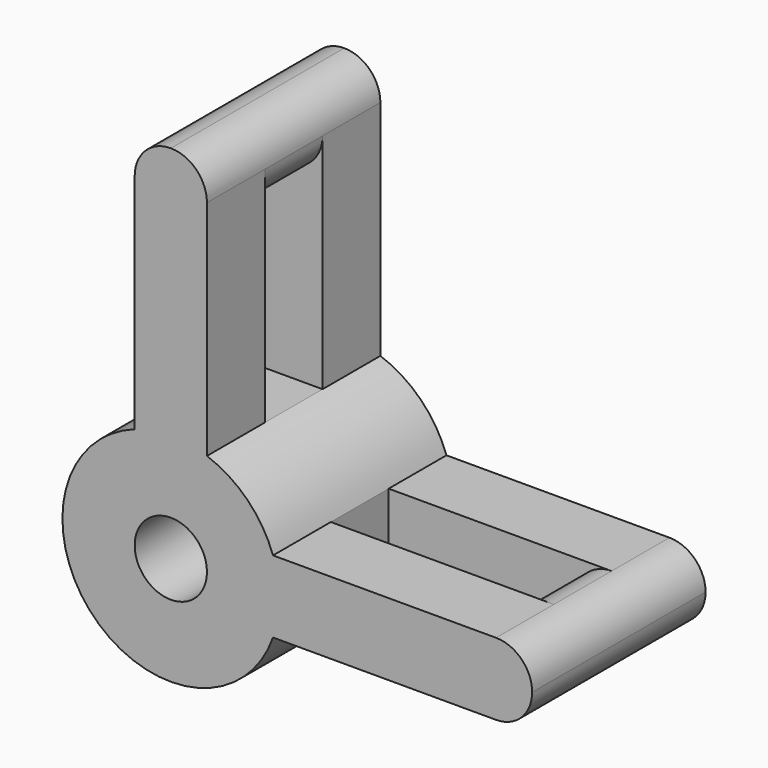
from build123d import *

# Parameters (mm, degrees)
F1_DEPTH = 15
F2_W     = 5
F2_H     = 12.9289321881
F3_DEPTH = 25
F4_W     = 12.9289321881
F4_H     = 5
F5_DEPTH = 25
F6_R     = 2.49999
F7_R     = 2.5
F8_DEPTH = 25


# Not quite as in the source:
# - a fillet or chamfer is up to 0.001 mm smaller than in the source, because OpenCascade refuses the exact size


with BuildPart() as f1:
    # F0 (on Front) → F1 (new body)
    with BuildSketch(Plane.XZ):
        with BuildLine():
            Line((2.5, 25), (-2.5, 25))
            Line((-2.5, 25), (-2.5, 7.0710678119))
            ThreePointArc((-2.5, 7.0710678119), (-5.3033008589, -5.3033008589), (7.0710678119, -2.5))
            Line((7.0710678119, -2.5), (25, -2.5))
            Line((25, -2.5), (25, 2.5))
            Line((25, 2.5), (7.0710678119, 2.5))
            ThreePointArc((7.0710678119, 2.5), (5.3033008589, 5.3033008589), (2.5, 7.0710678119))
            Line((2.5, 7.0710678119), (2.5, 25))
        make_face()
    extrude(amount=F1_DEPTH)

    # F2 (on face) → F3 (cut)
    with BuildSketch(Plane.YZ.offset(2.5)):
        with Locations((-7.5, 13.5355339059)):
            Rectangle(F2_W, F2_H)
    extrude(amount=-F3_DEPTH, mode=Mode.SUBTRACT)

    # F4 (on face) → F5 (cut)
    with BuildSketch(Plane.XY.offset(2.5)):
        with Locations((13.5355339059, -7.5)):
            Rectangle(F4_W, F4_H)
    extrude(amount=-F5_DEPTH, mode=Mode.SUBTRACT)

    # F6 (radius 2.5 in the source; OpenCascade refuses exactly that, so slightly less here)
    f6_edges = [f1.edges().sort_by_distance(p)[0] for p in [
        (-2.5, -7.5, 25),
        (2.5, -7.5, 25),
        (-2.5, -7.5, 20),
        (2.5, -7.5, 20),
        (25, -7.5, -2.5),
        (25, -7.5, 2.5),
        (20, -7.5, -2.5),
        (20, -7.5, 2.5),
    ]]
    fillet(f6_edges, radius=F6_R)

    # F7 (on face) → F8 (cut)
    with BuildSketch(Plane.XZ.offset(15)):
        Circle(F7_R)
    extrude(amount=-F8_DEPTH, mode=Mode.SUBTRACT)


solid = f1.part
